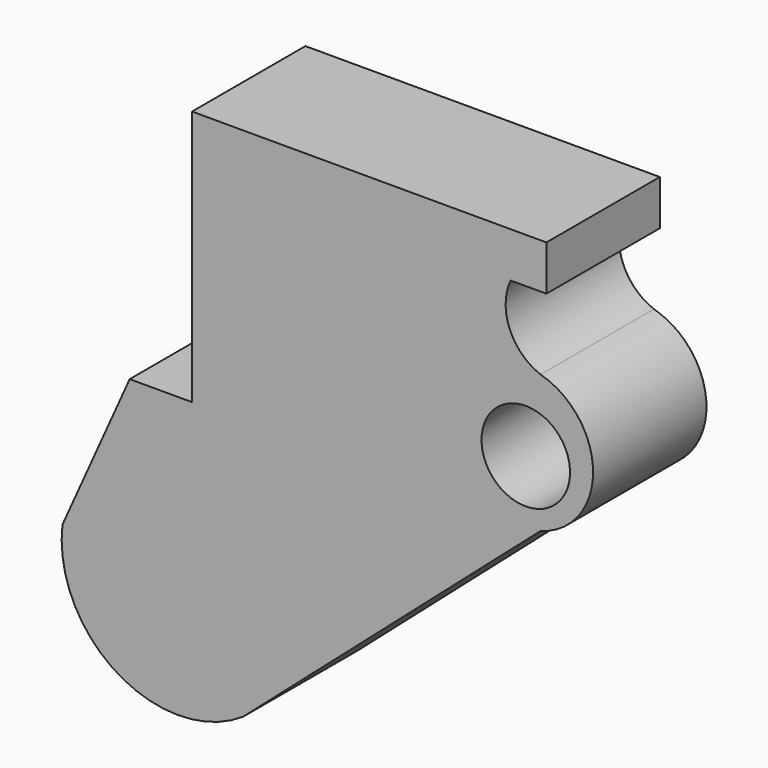
from build123d import *

# Parameters (mm, degrees)
F1_DEPTH = 2.54
F2_D     = 1.5875


# Not quite as in the source:
# - a feature names something its author has since deleted; it is built from what else it names


with BuildPart() as f1:
    # F0 (on Front) → F1 (new body)
    with BuildSketch(Plane.XZ):
        with BuildLine():
            Line((-49.06217859, 61.4019967616), (-49.06217859, 56.8155013025))
            Line((-49.06217859, 56.8155013025), (-42.814206332, 56.8155013025))
            ThreePointArc((-42.814206332, 56.8155013025), (-41.8729112238, 58.0492764711), (-42.814206332, 59.2830516398))
            ThreePointArc((-42.814206332, 59.2830516398), (-43.3685164044, 59.8206001728), (-43.3524362743, 60.592584312))
            Line((-43.3524362743, 60.592584312), (-42.7099727094, 60.592584312))
            Line((-42.7099727094, 60.592584312), (-42.7099727094, 61.4019967616))
            Line((-42.7099727094, 61.4019967616), (-49.06217859, 61.4019967616))
        make_face()
        with BuildLine():
            Line((-49.06217859, 56.8155013025), (-50.180206332, 56.8155013025))
            Line((-50.180206332, 56.8155013025), (-51.3855293393, 54.1270449758))
            ThreePointArc((-51.3855293393, 54.1270449758), (-50.3996469968, 52.1018542735), (-48.1477119029, 52.148219198))
            Line((-48.1477119029, 52.148219198), (-42.814206332, 56.8155013025))
            Line((-42.814206332, 56.8155013025), (-49.06217859, 56.8155013025))
        make_face()
    extrude(amount=F1_DEPTH)

    # F2 (through all)
    with Locations(Plane(origin=(0, 0, 0), x_dir=(1, 0, 0), z_dir=(0, 1, 0))):
        with Locations((-43.0801697075, -57.9093620181)):
            Hole(F2_D / 2)


solid = f1.part
